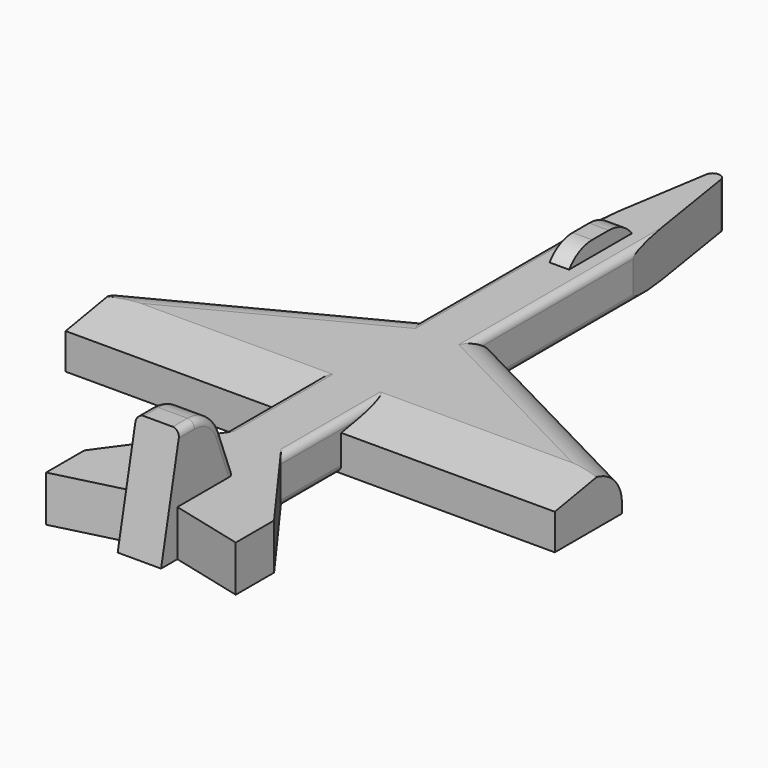
from build123d import *

# Parameters (mm, degrees)
F1_DEPTH      = 6.35
F2_W          = 1.3509193668
F2_H          = 10.8486381359
F3_DEPTH      = 2
F5_DEPTH      = 3
F7_R          = 5
F8_T1_DEPTH   = 22.7018387336
F9_T1_DEPTH   = 22.7018387336
F10_T1_DEPTH  = 37.7293119504
F11_T1_DEPTH  = 50.3092406281
F11_T3_DEPTH  = 50.3092406281
F11_T8_DEPTH  = 71.0975509994
F11_T13_DEPTH = 71.0975509994
F12_R         = 1
F13_R         = 1
F14_R         = 1
F15_R         = 1


# Not quite as in the source:
# - a fillet or chamfer that OpenCascade refuses, or shapes differently, is made with other operations: its cross-section is extruded or revolved along the edge and cut away or added


with BuildPart() as f1:
    # F0 (on Top) → F1 (new body)
    with BuildSketch(Plane.XY):
        Polygon((0, -66.0772249103), (0, 35.7286036015), (-4.0004998446, 10.6220170856), (-4.0004998446, -13.1050860509), (-33.7973274291, -28.5552926362), (-33.7973274291, -40.1429459453), (-4.2763971724, -40.1429459453), (-4.2763971724, -50.6270192564), (-13.1050860509, -62.766470015), (-13.1050860509, -69.3879872561), align=None)
    extrude(amount=F1_DEPTH)

    # F2 (on face) → F3 (join)
    with BuildSketch(Plane.XY.offset(6.35)):
        with Locations((-0.6754596834, 8.3060876932)):
            Rectangle(F2_W, F2_H)
    extrude(amount=F3_DEPTH)

    # F4 (on Right) → F5 (join)
    with BuildSketch(Plane.YZ):
        with BuildLine():
            Line((-69.653019309, 0), (-54.4461198151, 0))
            Line((-54.4461198151, 0), (-59.1908343158, 12.4009543867))
            ThreePointArc((-59.1908343158, 12.4009543867), (-61.0264090525, 14.733305135), (-63.8606947699, 15.6142245978))
            Line((-63.8606947699, 15.6142245978), (-66.3944035769, 15.6142245978))
            Line((-66.3944035769, 15.6142245978), (-69.653019309, 0))
        make_face()
    extrude(amount=-F5_DEPTH)

    # F6: F1 across face


with BuildPart() as f1_1:
    add(f1.part)
    add(f1.part.mirror(Plane(origin=(0, -20.6881401181, 4.0270783), x_dir=(0, 1, 0), z_dir=(1, 0, 0))))

    # F7
    f7_edges = [f1_1.edges().sort_by_distance(p)[0] for p in [
        (-18.898914, -20.830189, 6.35),
        (18.898914, -20.830189, 6.35),
    ]]
    fillet(f7_edges, radius=F7_R)

    # F8: fillet of radius 5 on 1 edges, made by hand

    # F8_s2 → F8_t1 (cut)
    with BuildSketch(Plane.YZ.offset(-11.3509193668)):
        with BuildLine():
            ThreePointArc((13.7304067612, 6.35), (11.9664747387, 7.822135955), (9.7304067612, 8.35))
            Line((9.7304067612, 8.35), (13.7304067612, 8.35))
            Line((13.7304067612, 8.35), (13.7304067612, 6.35))
        make_face()
    extrude(amount=F8_T1_DEPTH, mode=Mode.SUBTRACT)

    # F9: fillet of radius 5 on 1 edges, made by hand

    # F9_s2 → F9_t1 (cut)
    with BuildSketch(Plane.YZ.offset(-11.3509193668)):
        with BuildLine():
            ThreePointArc((2.8817686252, 6.35), (4.6457006477, 7.822135955), (6.8817686252, 8.35))
            Line((6.8817686252, 8.35), (2.8817686252, 8.35))
            Line((2.8817686252, 8.35), (2.8817686252, 6.35))
        make_face()
    extrude(amount=F9_T1_DEPTH, mode=Mode.SUBTRACT)

    # F10: fillet of radius 1 on 1 edges, made by hand

    # F10_s2 → F10_t1 (cut)
    with BuildSketch(Plane.XY.offset(-15.6896559752)):
        with BuildLine():
            ThreePointArc((-0.9875420089, 29.5309258493), (0, 30.3735702625), (0.9875420089, 29.5309258493))
            Line((0.9875420089, 29.5309258493), (0, 35.7286036015))
            Line((0, 35.7286036015), (-0.9875420089, 29.5309258493))
        make_face()
    extrude(amount=F10_T1_DEPTH, mode=Mode.SUBTRACT)

    # F11: chamfer of 8 x 1.4106158457 on 2 edges, made by hand

    # F11_s2 → F11_t1 (cut)
    with BuildSketch(Plane.YZ.offset(-54.5856378004)):
        Polygon((-32.1429459453, 6.35), (-40.1429459453, 4.9393841543), (-40.1429459453, 6.35), align=None)
    extrude(amount=F11_T1_DEPTH, mode=Mode.SUBTRACT)

    # F11_s4 → F11_t3 (cut)
    with BuildSketch(Plane.YZ.offset(4.2763971724)):
        Polygon((-32.1429459453, 6.35), (-40.1429459453, 4.9393841543), (-40.1429459453, 6.35), align=None)
    extrude(amount=F11_T3_DEPTH, mode=Mode.SUBTRACT)


with BuildPart() as f11_tool6:
    # F11_s7 → F11_t8 (new body)
    with BuildSketch(Plane.YZ.offset(-54.5856378004)):
        Polygon((-32.1429459453, 6.35), (-40.1429459453, 4.9393841543), (-40.1429459453, 6.35), align=None)
    extrude(amount=F11_T8_DEPTH)

    split(bisect_by=Plane.YZ.offset(4.2763971724), keep=Keep.TOP)


with BuildPart() as f1_2:
    add(f1_1.part)

    # F11_t5: cut F11_tool6
    add(f11_tool6.part, mode=Mode.SUBTRACT)


with BuildPart() as f11_tool11:
    # F11_s12 → F11_t13 (new body)
    with BuildSketch(Plane.YZ.offset(54.5856378004)):
        Polygon((-32.1429459453, 6.35), (-40.1429459453, 4.9393841543), (-40.1429459453, 6.35), align=None)
    extrude(amount=-F11_T13_DEPTH)

    split(bisect_by=Plane.YZ.offset(-4.2763971724), keep=Keep.BOTTOM)


with BuildPart() as f1_3:
    add(f1_2.part)

    # F11_t10: cut F11_tool11
    add(f11_tool11.part, mode=Mode.SUBTRACT)

    # F12
    f12_edges = [f1_3.edges().sort_by_distance(p)[0] for p in [
        (-3, -58.03326, 9.375477),
    ]]
    fillet(f12_edges, radius=F12_R)

    # F13
    f13_edges = [f1_3.edges().sort_by_distance(p)[0] for p in [
        (3, -58.03326, 9.375477),
    ]]
    fillet(f13_edges, radius=F13_R)

    # F14
    f14_edges = [f1_3.edges().sort_by_distance(p)[0] for p in [
        (4.0005, -4.057628, 6.35),
        (-4.0005, -4.057628, 6.35),
        (-4.276397, -41.384983, 6.35),
        (4.276397, -41.384983, 6.35),
    ]]
    fillet(f14_edges, radius=F14_R)

    # F15
    f15_edges = [f1_3.edges().sort_by_distance(p)[0] for p in [
        (4.0005, -1.241534, 0),
        (-4.0005, -1.241534, 0),
        (4.276397, -45.384983, 0),
    ]]
    fillet(f15_edges, radius=F15_R)


solid = f1_3.part
